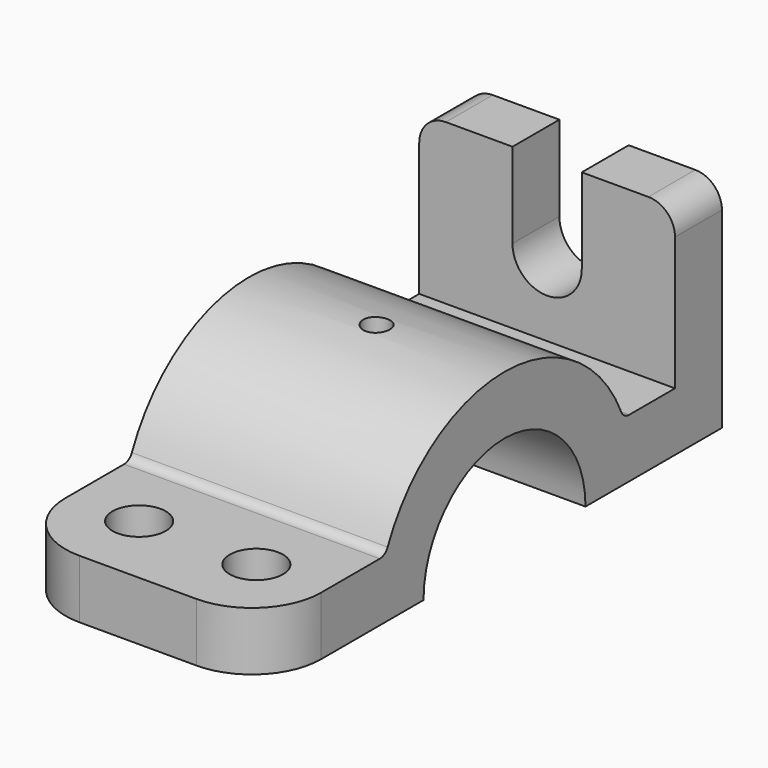
from build123d import *

# Parameters (mm, degrees)
F0_W     = 11
F0_H     = 30
F1_DEPTH = 24
F3_DEPTH = 11
F4_R     = 2.5
F4_R_2   = 5
F5_DEPTH = 41.001
F6_R     = 13
F7_R     = 5
F8_R     = 2


# Not quite as in the source:
# - a feature names something its author has since deleted; it is built from what else it names


with BuildPart() as f1:
    # F0 (on Right) → F1 (new body, symmetric)
    with BuildSketch(Plane.YZ):
        with BuildLine():
            ThreePointArc((15.4919333848, 11), (18.1017503893, 5.7729223833), (19, 0))
            Line((19, 0), (30, 0))
            ThreePointArc((30, 0), (29.4730143031, 5.5983415304), (27.9105714739, 11))
            Line((27.9105714739, 11), (15.4919333848, 11))
        make_face()
        with BuildLine():
            ThreePointArc((-15.4919333848, 11), (0, 19), (15.4919333848, 11))
            Line((15.4919333848, 11), (27.9105714739, 11))
            ThreePointArc((27.9105714739, 11), (0, 30), (-27.9105714739, 11))
            Line((-27.9105714739, 11), (-15.4919333848, 11))
        make_face()
        with BuildLine():
            Line((-30, 0), (-19, 0))
            ThreePointArc((-19, 0), (-18.1017503893, 5.7729223833), (-15.4919333848, 11))
            Line((-15.4919333848, 11), (-27.9105714739, 11))
            ThreePointArc((-27.9105714739, 11), (-29.4730143031, 5.5983415304), (-30, 0))
        make_face()
        with BuildLine():
            ThreePointArc((27.9105714739, 11), (29.4730143031, 5.5983415304), (30, 0))
            Line((30, 0), (51, 0))
            Line((51, 0), (51, 11))
            Line((51, 11), (40, 11))
            Line((40, 11), (27.9105714739, 11))
        make_face()
        with BuildLine():
            Line((-56, 0), (-30, 0))
            ThreePointArc((-30, 0), (-29.4730143031, 5.5983415304), (-27.9105714739, 11))
            Line((-27.9105714739, 11), (-56, 11))
            Line((-56, 11), (-56, 0))
        make_face()
        with Locations((45.5, 26)):
            Rectangle(F0_W, F0_H)
    extrude(amount=F1_DEPTH, both=True)

    # F2 (on face) → F3 (cut, through all)
    with BuildSketch(Plane(origin=(0, 51, 0), x_dir=(-1, 0, 0), z_dir=(0, 1, 0))):
        with BuildLine():
            ThreePointArc((-6.5, 25), (0, 18.5), (6.5, 25))
            ThreePointArc((6.5, 25), (0, 31.5), (-6.5, 25))
        make_face()
        with BuildLine():
            ThreePointArc((-6.5, 25), (0, 31.5), (6.5, 25))
            Line((6.5, 25), (6.5, 41))
            Line((6.5, 41), (-6.5, 41))
            Line((-6.5, 41), (-6.5, 25))
        make_face()
    extrude(amount=-F3_DEPTH, mode=Mode.SUBTRACT)

    # F4 (on Top) → F5 (cut, through all)
    with BuildSketch(Plane.XY):
        Circle(F4_R)
        with Locations((-11, -41.955285737)):
            Circle(F4_R_2)
        with Locations((11, -41.955285737)):
            Circle(F4_R_2)
    extrude(amount=F5_DEPTH, mode=Mode.SUBTRACT)

    # F6
    f6_edges = [f1.edges().sort_by_distance(p)[0] for p in [
        (24, -56, 5.5),
        (-24, -56, 5.5),
    ]]
    fillet(f6_edges, radius=F6_R)

    # F7
    f7_edges = [f1.edges().sort_by_distance(p)[0] for p in [
        (24, 45.5, 41),
        (-24, 45.5, 41),
    ]]
    fillet(f7_edges, radius=F7_R)

    # F8
    f8_edges = [f1.edges().sort_by_distance(p)[0] for p in [
        (0, -27.910571, 11),
        (0, 27.910571, 11),
    ]]
    fillet(f8_edges, radius=F8_R)


solid = f1.part
